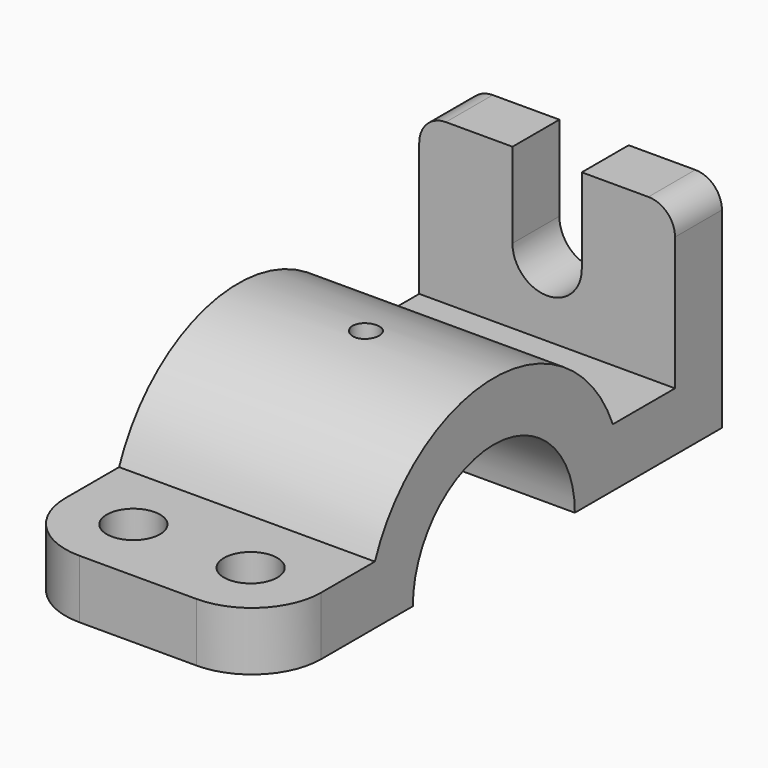
from build123d import *

# Parameters (mm, degrees)
F1_DEPTH = 24
F3_R     = 13
F4_R     = 5
F6_DEPTH = 11
F5_R     = 5
F5_R_2   = 2.5
F7_DEPTH = 41.001


# Not quite as in the source:
# - a feature names something its author has since deleted; it is built from what else it names


with BuildPart() as f1:
    # F0 (on Right) → F1 (new body, symmetric)
    with BuildSketch(Plane.YZ):
        with BuildLine():
            ThreePointArc((-19, 0), (0, 19), (19, 0))
            Line((19, 0), (53.5, 0))
            Line((53.5, 0), (53.5, 11))
            Line((53.5, 11), (53.5, 41))
            Line((53.5, 41), (42.5, 41))
            Line((42.5, 41), (42.5, 11))
            Line((42.5, 11), (27.9105714739, 11))
            ThreePointArc((27.9105714739, 11), (0, 30), (-27.9105714739, 11))
            Line((-27.9105714739, 11), (-53.5, 11))
            Line((-53.5, 11), (-53.5, 0))
            Line((-53.5, 0), (-19, 0))
        make_face()
    extrude(amount=F1_DEPTH, both=True)

    # F3
    f3_edges = [f1.edges().sort_by_distance(p)[0] for p in [
        (-24, -53.5, 5.5),
        (24, -53.5, 5.5),
    ]]
    fillet(f3_edges, radius=F3_R)

    # F4
    f4_edges = [f1.edges().sort_by_distance(p)[0] for p in [
        (-24, 48, 41),
        (24, 48, 41),
    ]]
    fillet(f4_edges, radius=F4_R)

    # F2 (on face) → F6 (cut, through all)
    with BuildSketch(Plane(origin=(0, 53.5, 0), x_dir=(-1, 0, 0), z_dir=(0, 1, 0))):
        with BuildLine():
            Line((-6.4999038836, 41), (-6.4999038836, 25.03534832))
            ThreePointArc((-6.4999038836, 25.03534832), (0.0014145677, 18.5000001539), (6.4998878825, 25.0381774101))
            Line((6.4998878825, 25.0381774101), (6.4998878825, 41))
            Line((6.4998878825, 41), (-6.4999038836, 41))
        make_face()
    extrude(amount=-F6_DEPTH, mode=Mode.SUBTRACT)

    # F5 (on Top) → F7 (cut, through all)
    with BuildSketch(Plane.XY):
        with Locations((-11, -40.7964820042)):
            Circle(F5_R)
        with Locations((11, -40.7964820042)):
            Circle(F5_R)
        Circle(F5_R_2)
    extrude(amount=F7_DEPTH, mode=Mode.SUBTRACT)


solid = f1.part
